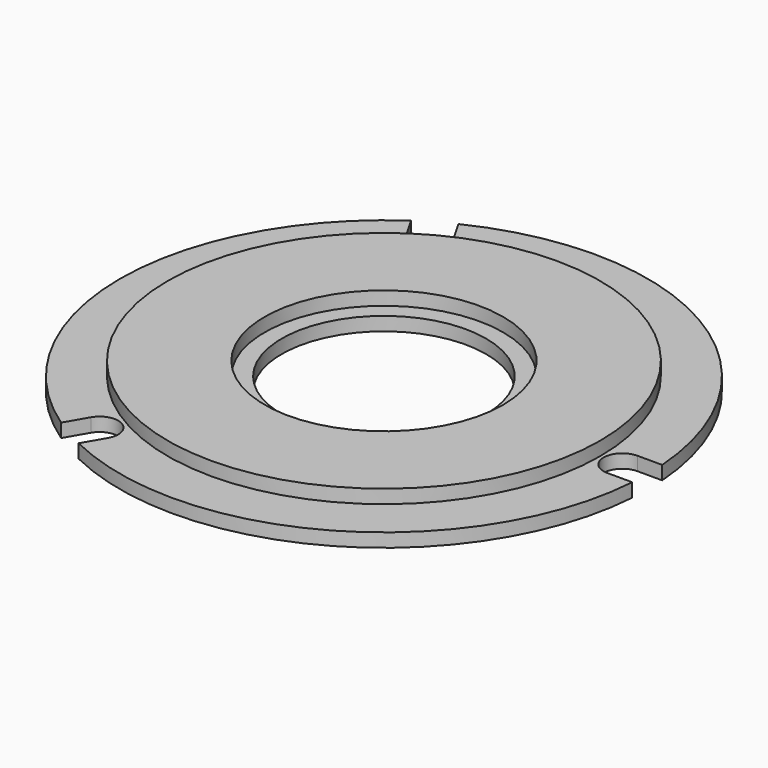
from build123d import *

# Parameters (mm, degrees)
F0_R            = 30
F1_DEPTH        = 4
F2_DEPTH        = 25
F2_COPIES_COUNT = 3
F4_R            = 63.5
F4_R_2          = 35
F5_DEPTH        = 4


# Not quite as in the source:
# - a pattern or mirror of a feature is missing from the dataset's text; its kind, count and spacing are read off the source's solid


with BuildPart() as f1:
    # F0 (on Top) → F1 (new body)
    with BuildSketch(Plane.XY):
        with BuildLine():
            Line((70, 5.5), (77.3045923604, 5.5))
            ThreePointArc((77.3045923604, 5.5), (-77.5, 0), (77.3045923604, -5.5))
            Line((77.3045923604, -5.5), (70, -5.5))
            ThreePointArc((70, -5.5), (64.5, 0), (70, 5.5))
        make_face()
        Circle(F0_R, mode=Mode.SUBTRACT)
        with BuildLine():
            ThreePointArc((77.3045923604, -5.5), (77.4511326835, -2.7517350956), (77.5, 0))
            ThreePointArc((77.5, 0), (77.4511326835, 2.7517350956), (77.3045923604, 5.5))
            Line((77.3045923604, 5.5), (70, 5.5))
            ThreePointArc((70, 5.5), (73.8890872965, 3.8890872965), (75.5, 0))
            ThreePointArc((75.5, 0), (73.8890872965, -3.8890872965), (70, -5.5))
            Line((70, -5.5), (77.3045923604, -5.5))
        make_face()
        with BuildLine():
            ThreePointArc((75.5, 0), (73.8890872965, 3.8890872965), (70, 5.5))
            ThreePointArc((70, 5.5), (64.5, 0), (70, -5.5))
            ThreePointArc((70, -5.5), (73.8890872965, -3.8890872965), (75.5, 0))
        make_face()
    extrude(amount=F1_DEPTH)

    # F0 (on Top) → F2 (cut)
    with BuildSketch(Plane.XY):
        with BuildLine():
            ThreePointArc((75.5, 0), (73.8890872965, 3.8890872965), (70, 5.5))
            ThreePointArc((70, 5.5), (64.5, 0), (70, -5.5))
            ThreePointArc((70, -5.5), (73.8890872965, -3.8890872965), (75.5, 0))
        make_face()
        with BuildLine():
            ThreePointArc((77.3045923604, -5.5), (77.4511326835, -2.7517350956), (77.5, 0))
            ThreePointArc((77.5, 0), (77.4511326835, 2.7517350956), (77.3045923604, 5.5))
            Line((77.3045923604, 5.5), (70, 5.5))
            ThreePointArc((70, 5.5), (73.8890872965, 3.8890872965), (75.5, 0))
            ThreePointArc((75.5, 0), (73.8890872965, -3.8890872965), (70, -5.5))
            Line((70, -5.5), (77.3045923604, -5.5))
        make_face()
    f2 = extrude(amount=F2_DEPTH, mode=Mode.SUBTRACT)

    # F2_copies: F2 ×3 about axis
    f2_copies_axis = Axis((0, 0, 0), (0, 0, 1))
    for i in range(1, F2_COPIES_COUNT):
        add(f2.rotate(f2_copies_axis, i * 360 / F2_COPIES_COUNT), mode=Mode.SUBTRACT)


with BuildPart() as f5:
    # F4 (on face) → F5 (new body)
    with BuildSketch(Plane.XY.offset(4)):
        Circle(F4_R)
        Circle(F4_R_2, mode=Mode.SUBTRACT)
    extrude(amount=F5_DEPTH)


solid = Compound([f1.part, f5.part])
